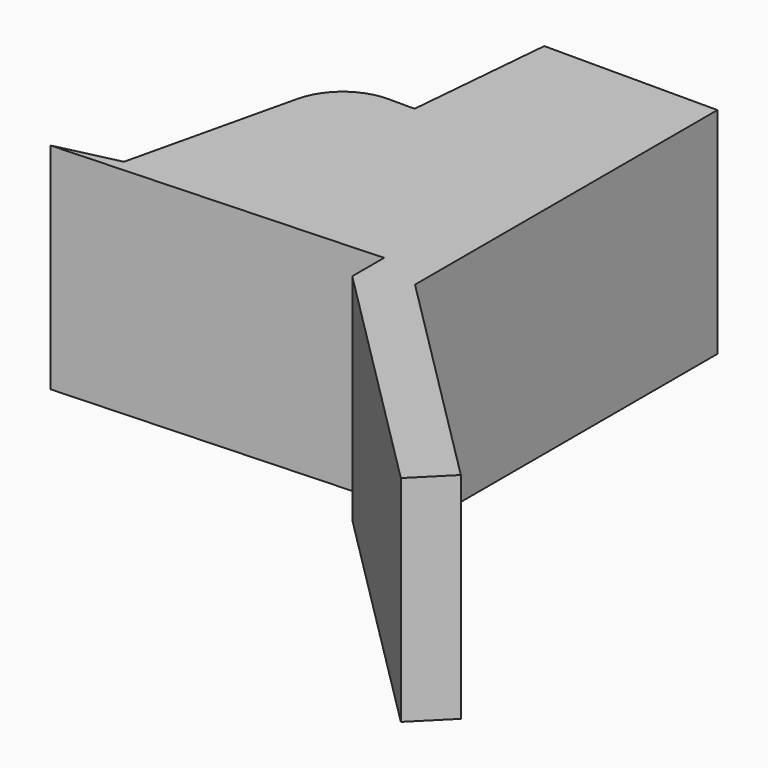
from build123d import *

# Parameters (mm, degrees)
F1_DEPTH      = 15
F4_DEPTH      = 9.2
F4_DEPTH_BACK = 1
F7_DEPTH      = 1.5
F8_SIZE       = 1.49999
F9_R          = 5
F11_DEPTH     = 4
F12_T4_DEPTH  = 6.4753623201
F12_S5_R      = 22.299103121
F12_T6_DEPTH  = 5
F12_S8_R      = 5
F12_T9_DEPTH  = 5
F12_T13_DEPTH = 6.4753623415
F12_S15_R     = 5
F12_T16_DEPTH = 5
F12_S17_R     = 22.299103121
F12_T18_DEPTH = 5


# Not quite as in the source:
# - a fillet or chamfer that OpenCascade refuses, or shapes differently, is made with other operations: its cross-section is extruded or revolved along the edge and cut away or added
# - a fillet or chamfer is up to 0.001 mm smaller than in the source, because OpenCascade refuses the exact size


with BuildPart() as f1:
    # F0 (on Top) → F1 (new body)
    with BuildSketch(Plane.XY):
        with BuildLine():
            Line((37.0060966544, -19.4203102168), (21, -3.4142135624))
            Line((21, -3.4142135624), (21, 23))
            Line((21, 23), (8.9, 23))
            Line((8.9, 23), (8.0008047996, 12.8091210619))
            ThreePointArc((8.0008047996, 12.8091210619), (7.9975966714, 12.8026247244), (7.9908435011, 12.8))
            Line((7.9908435011, 12.8), (6.1708946074, 12.8))
            ThreePointArc((6.1708946074, 12.8), (3.6860466407, 11.9345702389), (2.2764293651, 9.7127652912))
            Line((2.2764293651, 9.7127652912), (-0.46875, -2))
            Line((-0.46875, -2), (-4.7960747033, -3))
            Line((-4.7960747033, -3), (17.7071067812, -2))
            Line((17.7071067812, -2), (17.7071067812, -4.7781745931))
            Line((17.7071067812, -4.7781745931), (34.6776695297, -21.7487373415))
            Line((34.6776695297, -21.7487373415), (37.0060966544, -19.4203102168))
        make_face()
    extrude(amount=F1_DEPTH)

    # F3 (on face) → F4 (cut, two sides)
    with BuildSketch(Plane(origin=(2.0824892704, 23.6015450644, 0), x_dir=(0.99612985, -0.0878938103, 0), z_dir=(-0.0878938103, -0.99612985, 0))) as f4_sk:
        with BuildLine():
            Line((6.8439980284, 15), (6.8439980284, 0))
            ThreePointArc((6.8439980284, 0), (8.1431011494, 7.5), (6.8439980284, 15))
        make_face()
    extrude(amount=F4_DEPTH, mode=Mode.SUBTRACT)
    extrude(f4_sk.sketch, amount=-F4_DEPTH_BACK, mode=Mode.SUBTRACT)

    # F6 (on offset) → F7 (join)
    with BuildSketch(Plane(origin=(0, 23, 0), x_dir=(-1, 0, 0), z_dir=(0, 1, 0))):
        with BuildLine():
            ThreePointArc((-7.0033527857, 9.4235612132), (-7.0960699027, 7.4999998768), (-7.0033527857, 5.5764385404))
            Line((-7.0033527857, 5.5764385404), (-5.4957957644, 5.5764385404))
            ThreePointArc((-5.4957957644, 5.5764385404), (-5.5960699027, 7.4999998768), (-5.4957957644, 9.4235612132))
            Line((-5.4957957644, 9.4235612132), (-7.0033527857, 9.4235612132))
        make_face()
        with BuildLine():
            Line((-14.0960699027, 7.4999998768), (-14.0960699027, 5.5764385404))
            Line((-14.0960699027, 5.5764385404), (-7.0033527857, 5.5764385404))
            ThreePointArc((-7.0033527857, 5.5764385404), (-7.0960699027, 7.4999998768), (-7.0033527857, 9.4235612132))
            Line((-7.0033527857, 9.4235612132), (-14.0960699027, 9.4235612132))
            Line((-14.0960699027, 9.4235612132), (-14.0960699027, 7.4999998768))
        make_face()
    extrude(amount=F7_DEPTH)

    # F8 (size 1.5 in the source; OpenCascade refuses exactly that, so slightly less here)
    f8_edges = [f1.edges().sort_by_distance(p)[0] for p in [
        (14.09607, 24.5, 7.5),
    ]]
    chamfer(f8_edges, length=F8_SIZE)

    # F9
    f9_edges = [f1.edges().sort_by_distance(p)[0] for p in [
        (12.59608, 24.5, 7.5),
    ]]
    fillet(f9_edges, radius=F9_R)

    # F10 (on face) → F11 (cut)
    with BuildSketch(Plane.XY.offset(9.4235612132)):
        Polygon((5.4957957644, 22), (6.5002299745, 22), (5.4957957644, 24.5), align=None)
    extrude(amount=-F11_DEPTH, mode=Mode.SUBTRACT)

    # F12: fillet of radius 1 on 3 edges, made by hand


with BuildPart() as f12_tool2:
    # F12_s3 → F12_t4 (new body)
    with BuildSketch(Plane.YZ.offset(7.6207075826)):
        with BuildLine():
            ThreePointArc((23, 10.4235612132), (23.2928932188, 9.716454432), (24, 9.4235612132))
            Line((24, 9.4235612132), (24, 9.4035612132))
            Line((24, 9.4035612132), (22.98, 9.4035612132))
            Line((22.98, 9.4035612132), (22.98, 10.4235612132))
            Line((22.98, 10.4235612132), (23, 10.4235612132))
        make_face()
    extrude(amount=F12_T4_DEPTH)

    # F12_s5 → F12_t6 (cut, symmetric)
    with BuildSketch(Plane(origin=(2.1446089712, 24.3055683406, 0), x_dir=(0, 0, 1), z_dir=(0.0878938103, 0.99612985, 0))):
        with Locations((7.5, -14.1560019716)):
            Circle(F12_S5_R)
    extrude(amount=F12_T6_DEPTH, both=True, mode=Mode.SUBTRACT)

    split(bisect_by=Plane.XZ.offset(-23), keep=Keep.BOTTOM)

    # F12_s8 → F12_t9 (intersect, symmetric)
    with BuildSketch(Plane.XY.offset(9.9)):
        with Locations((10.5250120908, 19.5)):
            Circle(F12_S8_R)
    extrude(amount=F12_T9_DEPTH, both=True, mode=Mode.INTERSECT)


with BuildPart() as f1_1:
    add(f1.part)

    # F12_t1: union F12_tool2
    add(f12_tool2.part)


with BuildPart() as f12_tool11:
    # F12_s12 → F12_t13 (new body)
    with BuildSketch(Plane.YZ.offset(14.0960699027)):
        with BuildLine():
            ThreePointArc((24, 5.5764385404), (23.2928932188, 5.2835453216), (23, 4.5764385404))
            Line((23, 4.5764385404), (22.98, 4.5764385404))
            Line((22.98, 4.5764385404), (22.98, 5.5964385404))
            Line((22.98, 5.5964385404), (24, 5.5964385404))
            Line((24, 5.5964385404), (24, 5.5764385404))
        make_face()
    extrude(amount=-F12_T13_DEPTH)

    split(bisect_by=Plane.XZ.offset(-23), keep=Keep.BOTTOM)

    # F12_s15 → F12_t16 (intersect, symmetric)
    with BuildSketch(Plane.XY.offset(5.1)):
        with Locations((10.5250120908, 19.5)):
            Circle(F12_S15_R)
    extrude(amount=F12_T16_DEPTH, both=True, mode=Mode.INTERSECT)

    # F12_s17 → F12_t18 (cut, symmetric)
    with BuildSketch(Plane(origin=(2.1446089712, 24.3055683406, 0), x_dir=(0, 0, 1), z_dir=(0.0878938103, 0.99612985, 0))):
        with Locations((7.5, -14.1560019716)):
            Circle(F12_S17_R)
    extrude(amount=F12_T18_DEPTH, both=True, mode=Mode.SUBTRACT)


with BuildPart() as f1_2:
    add(f1_1.part)

    # F12_t10: union F12_tool11
    add(f12_tool11.part)


solid = f1_2.part
